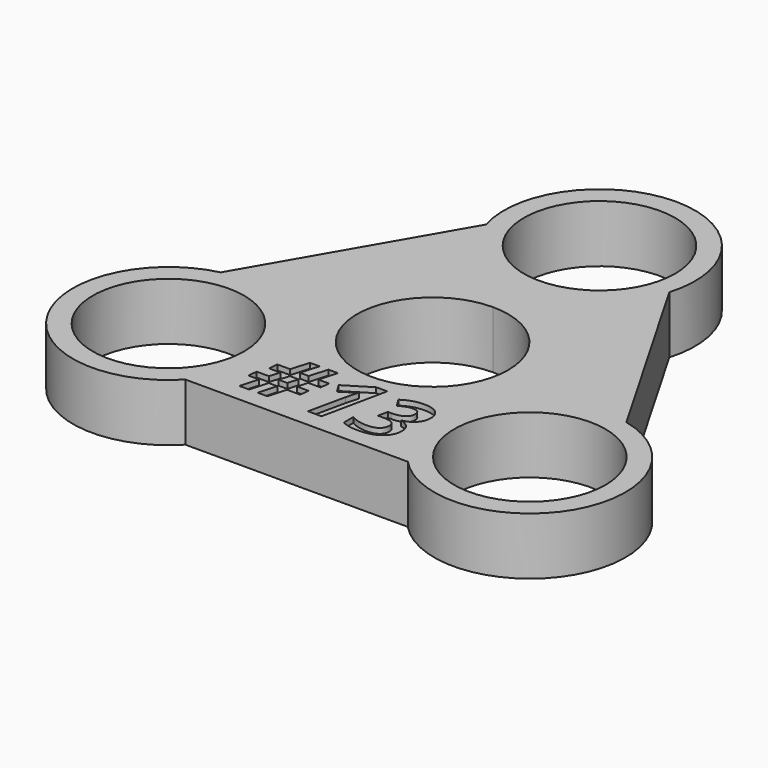
from build123d import *

# Parameters (mm, degrees)
F0_R         = 11.049
F1_DEPTH     = 8.382
F2_TEXT_SIZE = 13.3001400779
F3_DEPTH     = 0.762


# Not quite as in the source:
# - Text() gives the source's letters only with a copy of the font that has no kerning and outlines rounded to 1/6400 em; it was checked with that copy


with BuildPart() as f1:
    # F0 (on Top) → F1 (new body)
    with BuildSketch(Plane.XY):
        with BuildLine():
            Line((29.6332551726, -1.6459795066), (13.3883755138, 26.4909774253))
            ThreePointArc((13.3883755138, 26.4909774253), (-0.0002716343, 44.4499999974), (-13.3882203777, 26.4904567782))
            Line((-13.3882203777, 26.4904567782), (-29.6316081936, -1.6439162062))
            ThreePointArc((-29.6316081936, -1.6439162062), (-38.4951494341, -22.2140163886), (-16.2511343218, -24.8398832022))
            Line((-16.2511343218, -24.8398832022), (16.2479664191, -24.8398832022))
            ThreePointArc((16.2479664191, -24.8398832022), (38.4917451803, -22.2175492933), (29.6332551726, -1.6459795066))
        make_face()
        with Locations((-26.3964543073, -15.24)):
            Circle(F0_R, mode=Mode.SUBTRACT)
        with Locations((26.3964543073, -15.24)):
            Circle(F0_R, mode=Mode.SUBTRACT)
        with BuildLine():
            ThreePointArc((0, 11.049), (7.8128228253, 7.8128228253), (11.049, 0))
            ThreePointArc((11.049, 0), (-7.8128228253, -7.8128228253), (0, 11.049))
        make_face(mode=Mode.SUBTRACT)
        with Locations((0, 30.48)):
            Circle(F0_R, mode=Mode.SUBTRACT)
    extrude(amount=F1_DEPTH)

    # F2 (on face) → F3 (cut)
    with BuildSketch(Plane.XY.offset(8.382)):
        with Locations((-11.5034240298, -22.2251042724)):
            Text('#13', F2_TEXT_SIZE, font='Open Sans', font_style=FontStyle.BOLDITALIC, text_align=(TextAlign.LEFT, TextAlign.BOTTOM))
    extrude(amount=-F3_DEPTH, mode=Mode.SUBTRACT)


solid = f1.part
